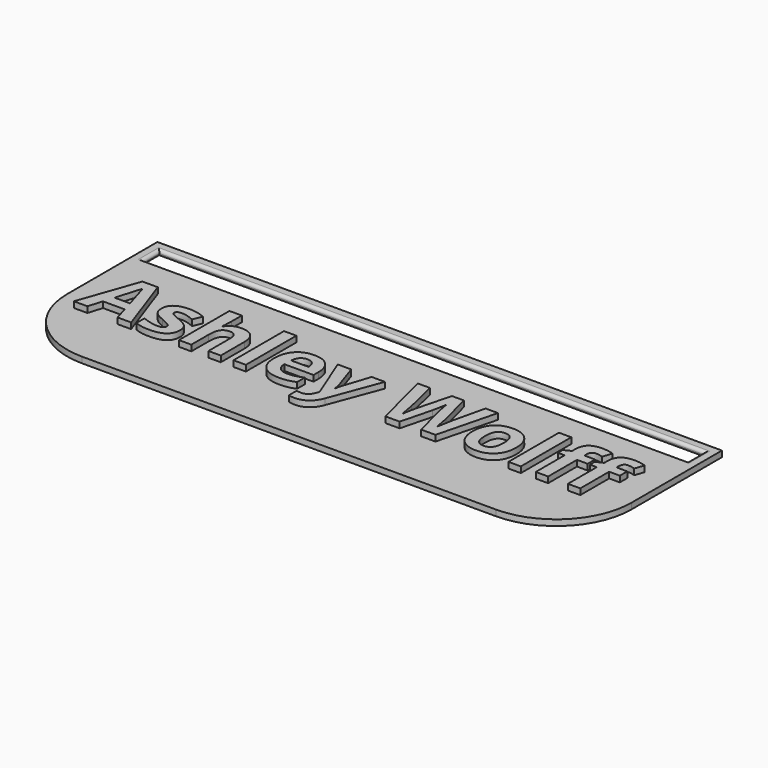
from build123d import *

# Parameters (mm, degrees)
F0_W         = 190.5
F0_H         = 63.5
F1_DEPTH     = 2
F2_W         = 183.896
F2_H         = 7.62
F3_DEPTH     = 25.4
F4_R         = 0.99999
F5_R         = 0.99999
F6_R         = 25.4
F7_TEXT_SIZE = 28.0248251404
F8_DEPTH     = 2


# Not quite as in the source:
# - a fillet or chamfer is up to 0.001 mm smaller than in the source, because OpenCascade refuses the exact size
# - Text() gives the source's letters only with a copy of the font that has no kerning and outlines rounded to 1/6400 em; it was checked with that copy


with BuildPart() as f1:
    # F0 (on Top) → F1 (new body)
    with BuildSketch(Plane.XY):
        with Locations((1.791532172, 31.75)):
            Rectangle(F0_W, F0_H)
    extrude(amount=F1_DEPTH)

    # F2 (on face) → F3 (cut)
    with BuildSketch(Plane.XY.offset(2)):
        with Locations((1.791532172, 56.388)):
            Rectangle(F2_W, F2_H)
    extrude(amount=-F3_DEPTH, mode=Mode.SUBTRACT)

    # F4 (radius 1 in the source; OpenCascade refuses exactly that, so slightly less here)
    f4_edges = [f1.edges().sort_by_distance(p)[0] for p in [
        (1.791532, 60.198, 2),
        (1.791532, 60.198, 0),
    ]]
    fillet(f4_edges, radius=F4_R)

    # F5 (radius 1 in the source; OpenCascade refuses exactly that, so slightly less here)
    f5_edges = [f1.edges().sort_by_distance(p)[0] for p in [
        (93.739532, 56.388, 0),
        (93.739532, 56.388, 2),
        (-90.156468, 56.388, 2),
        (-90.156468, 56.388, 0),
    ]]
    fillet(f5_edges, radius=F5_R)

    # F6
    f6_edges = [f1.edges().sort_by_distance(p)[0] for p in [
        (-93.458468, 0, 1),
        (97.041532, 0, 1),
    ]]
    fillet(f6_edges, radius=F6_R)

    # F7 (on face) → F8 (join)
    with BuildSketch(Plane.XY.offset(2)):
        with Locations((-87.108467828, 20.32)):
            Text('Ashley Wolff', F7_TEXT_SIZE, font='Open Sans', font_style=FontStyle.BOLD, text_align=(TextAlign.LEFT, TextAlign.BOTTOM))
    extrude(amount=F8_DEPTH)


solid = f1.part
